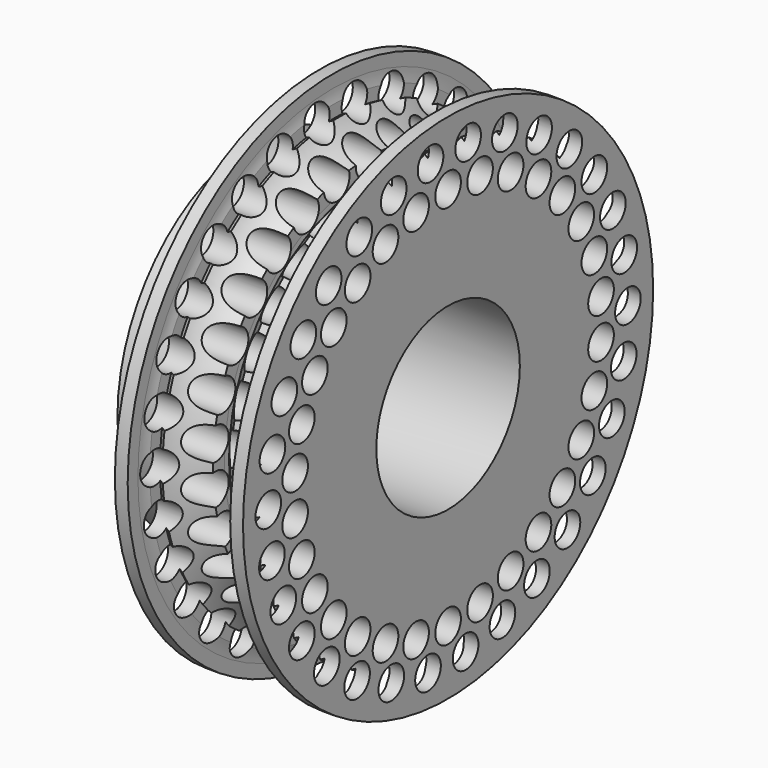
from build123d import *
from build123d import SkipClean  # not in build123d's __all__

# Parameters (mm, degrees)
F2_R     = 1.25
F3_DEPTH = 25
F4_R     = 13.5
F4_R_2   = 7
F5_DEPTH = 5


with BuildPart() as f1:
    # F0 (on Top) → F1 (revolve)
    with BuildSketch(Plane.XY):
        with BuildLine():
            Line((-2.1759010437, 20), (-2.1759010437, 7))
            Line((-2.1759010437, 7), (7.8240989563, 7))
            Line((7.8240989563, 7), (7.8240989563, 20))
            Line((7.8240989563, 20), (6.8240989563, 20))
            Line((6.8240989563, 20), (6.8240989563, 19))
            ThreePointArc((6.8240989563, 19), (6.7916377134, 18.491437112), (6.6947808508, 17.9911285158))
            Line((6.6947808508, 17.9911285158), (6.6947808508, 17.0031964998))
            Line((6.6947808508, 17.0031964998), (6.3751726346, 17.1588384831))
            ThreePointArc((6.3751726346, 17.1588384831), (5.3945982782, 15.9352759935), (4.0190295517, 15.1826526393))
            Line((4.0190295517, 15.1826526393), (4.0169301266, 13.6502641967))
            Line((4.0169301266, 13.6502641967), (2.8378947431, 15.0000237905))
            Line((2.8378947431, 15.0000237905), (1.6441955231, 13.6416424066))
            Line((1.6441955231, 13.6416424066), (1.6307138139, 14.0546131879))
            Line((1.6307138139, 14.0546131879), (1.629168361, 15.1826526393))
            ThreePointArc((1.629168361, 15.1826526393), (0.2535996345, 15.9352759935), (-0.726974722, 17.1588384831))
            Line((-0.726974722, 17.1588384831), (-1.0465829382, 17.0031964998))
            Line((-1.0465829382, 17.0031964998), (-1.0465829382, 17.9911285158))
            ThreePointArc((-1.0465829382, 17.9911285158), (-1.1434398008, 18.491437112), (-1.1759010437, 19))
            Line((-1.1759010437, 19), (-1.1759010437, 20))
            Line((-1.1759010437, 20), (-2.1759010437, 20))
        make_face()
    revolve(axis=Axis((6.8483626047, 0, 0), (1, 0, 0)))

    # F2 (on face) → F3 (cut)
    with BuildSketch(Plane.YZ.offset(7.8240989563)):
        with Locations((0, 15)):
            Circle(F2_R)
        with Locations((-8.8167787844, 12.1352549156)):
            Circle(F2_R)
        with Locations((-14.2658477444, 4.6352549156)):
            Circle(F2_R)
        with Locations((-14.2658477444, -4.6352549156)):
            Circle(F2_R)
        with Locations((-8.8167787844, -12.1352549156)):
            Circle(F2_R)
        with Locations((0, -15)):
            Circle(F2_R)
        with Locations((8.8167787844, -12.1352549156)):
            Circle(F2_R)
        with Locations((14.2658477444, -4.6352549156)):
            Circle(F2_R)
        with Locations((14.2658477444, 4.6352549156)):
            Circle(F2_R)
        with Locations((8.8167787844, 12.1352549156)):
            Circle(F2_R)
        with Locations((-6.1010496461, -13.7031818646)):
            Circle(F2_R)
        with Locations((6.1010496461, 13.7031818646)):
            Circle(F2_R)
        with Locations((-11.1471723822, 10.0369590954)):
            Circle(F2_R)
        with Locations((-3.1186753623, 14.672214011)):
            Circle(F2_R)
        with Locations((3.1186753623, -14.672214011)):
            Circle(F2_R)
        with Locations((11.1471723822, -10.0369590954)):
            Circle(F2_R)
        with Locations((12.9903810568, 7.5)):
            Circle(F2_R)
        with Locations((-12.9903810568, -7.5)):
            Circle(F2_R)
        with Locations((14.9178284305, -1.567926949)):
            Circle(F2_R)
        with Locations((-14.9178284305, 1.567926949)):
            Circle(F2_R)
        with Locations((14.9178284305, 1.567926949)):
            Circle(F2_R)
        with Locations((-14.9178284305, -1.567926949)):
            Circle(F2_R)
        with Locations((-3.1186753623, -14.672214011)):
            Circle(F2_R)
        with Locations((-11.1471723822, -10.0369590954)):
            Circle(F2_R)
        with Locations((11.1471723822, 10.0369590954)):
            Circle(F2_R)
        with Locations((3.1186753623, 14.672214011)):
            Circle(F2_R)
        with Locations((-12.9903810568, 7.5)):
            Circle(F2_R)
        with Locations((12.9903810568, -7.5)):
            Circle(F2_R)
        with Locations((-6.1010496461, 13.7031818646)):
            Circle(F2_R)
        with Locations((6.1010496461, -13.7031818646)):
            Circle(F2_R)
        with Locations((1.9566006958, 17.4308139831)):
            Circle(F2_R)
        with Locations((-8.6626521806, 15.2518857717)):
            Circle(F2_R)
        with Locations((-15.9730663567, 7.2472555881)):
            Circle(F2_R)
        with Locations((-17.1823120892, -3.525579905)):
            Circle(F2_R)
        with Locations((-11.8284986089, -12.9517637045)):
            Circle(F2_R)
        with Locations((-1.9566006958, -17.4308139831)):
            Circle(F2_R)
        with Locations((8.6626521806, -15.2518857717)):
            Circle(F2_R)
        with Locations((15.9730663567, -7.2472555881)):
            Circle(F2_R)
        with Locations((17.1823120892, 3.525579905)):
            Circle(F2_R)
        with Locations((11.8284986089, 12.9517637045)):
            Circle(F2_R)
        with Locations((-11.6443978054, 13.1175288125)):
            Circle(F2_R)
        with Locations((-17.1308056963, 3.7678984317)):
            Circle(F2_R)
        with Locations((-16.0738280659, -7.0209410839)):
            Circle(F2_R)
        with Locations((-8.8771944437, -15.1280197384)):
            Circle(F2_R)
        with Locations((1.7102257313, -17.4567090353)):
            Circle(F2_R)
        with Locations((11.6443978054, -13.1175288125)):
            Circle(F2_R)
        with Locations((17.1308056963, -3.7678984317)):
            Circle(F2_R)
        with Locations((16.0738280659, 7.0209410839)):
            Circle(F2_R)
        with Locations((8.8771944437, 15.1280197384)):
            Circle(F2_R)
        with Locations((-1.7102257313, 17.4567090353)):
            Circle(F2_R)
        with Locations((-5.5379142838, -16.6431087175)):
            Circle(F2_R)
        with Locations((5.3023070874, -16.7196621361)):
            Circle(F2_R)
        with Locations((14.1172273701, -10.4098728992)):
            Circle(F2_R)
        with Locations((17.5398466242, -0.1238660334)):
            Circle(F2_R)
        with Locations((14.2628406254, 10.2094534472)):
            Circle(F2_R)
        with Locations((5.5379142838, 16.6431087175)):
            Circle(F2_R)
        with Locations((-5.3023070874, 16.7196621361)):
            Circle(F2_R)
        with Locations((-14.1172273701, 10.4098728992)):
            Circle(F2_R)
        with Locations((-17.5398466242, 0.1238660334)):
            Circle(F2_R)
        with Locations((-14.2628406254, -10.2094534472)):
            Circle(F2_R)
    extrude(amount=-F3_DEPTH, mode=Mode.SUBTRACT)

    # F4 (on face) → F5 (join)
    with BuildSketch(Plane(origin=(-2.1759010437, 0, 0), x_dir=(0, -1, 0), z_dir=(-1, 0, 0))):
        Circle(F4_R)
        Circle(F4_R_2, mode=Mode.SUBTRACT)
    with SkipClean():  # cleaning this boolean's faces spoils the solid; the shape is the same uncleaned
        extrude(amount=F5_DEPTH)


solid = f1.part
